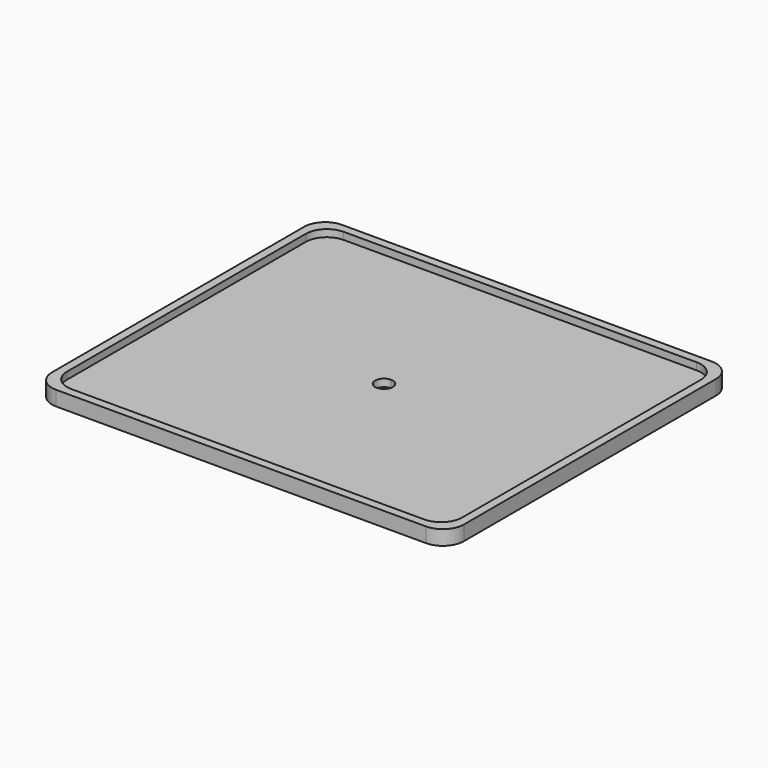
from build123d import *

# Parameters (mm, degrees)
F1_DEPTH = 1.8
F2_R     = 5
F3_DEPTH = 3.5
F4_R     = 5
F5_R     = 5


# Not quite as in the source:
# - a feature names something its author has since deleted; it is built from what else it names


with BuildPart() as f1:
    # F0 (on Top) → F1 (new body)
    with BuildSketch(Plane.XY):
        Polygon((-98, 0), (0, 0), (0, 85), (-49, 85), (-98, 85), align=None)
        Polygon((-96, 83), (-49, 83), (-2, 83), (-2, 2), (-96, 2), align=None, mode=Mode.SUBTRACT)
        Polygon((-2, 83), (-49, 83), (-96, 83), (-96, 2), (-2, 2), align=None)
        with BuildLine():
            ThreePointArc((-46.9, 42.5), (-50.4849242405, 41.0150757595), (-49, 44.6))
            ThreePointArc((-49, 44.6), (-47.5150757595, 43.9849242405), (-46.9, 42.5))
        make_face(mode=Mode.SUBTRACT)
    extrude(amount=F1_DEPTH)

    # F2
    f2_edges = [f1.edges().sort_by_distance(p)[0] for p in [
        (-98, 85, 0.9),
        (-98, 0, 0.9),
        (0, 0, 0.9),
        (0, 85, 0.9),
    ]]
    fillet(f2_edges, radius=F2_R)

    # F0 (on Top) → F3 (join)
    with BuildSketch(Plane.XY):
        Polygon((-98, 0), (0, 0), (0, 85), (-49, 85), (-98, 85), align=None)
        Polygon((-96, 83), (-49, 83), (-2, 83), (-2, 2), (-96, 2), align=None, mode=Mode.SUBTRACT)
    extrude(amount=F3_DEPTH)

    # F4
    f4_edges = [f1.edges().sort_by_distance(p)[0] for p in [
        (0, 85, 1.75),
        (0, 0, 1.75),
        (-98, 0, 1.75),
        (-98, 85, 1.75),
    ]]
    fillet(f4_edges, radius=F4_R)

    # F5
    f5_edges = [f1.edges().sort_by_distance(p)[0] for p in [
        (-96, 83, 2.65),
        (-96, 2, 2.65),
        (-2, 83, 2.65),
        (-2, 2, 2.65),
    ]]
    fillet(f5_edges, radius=F5_R)


solid = f1.part
